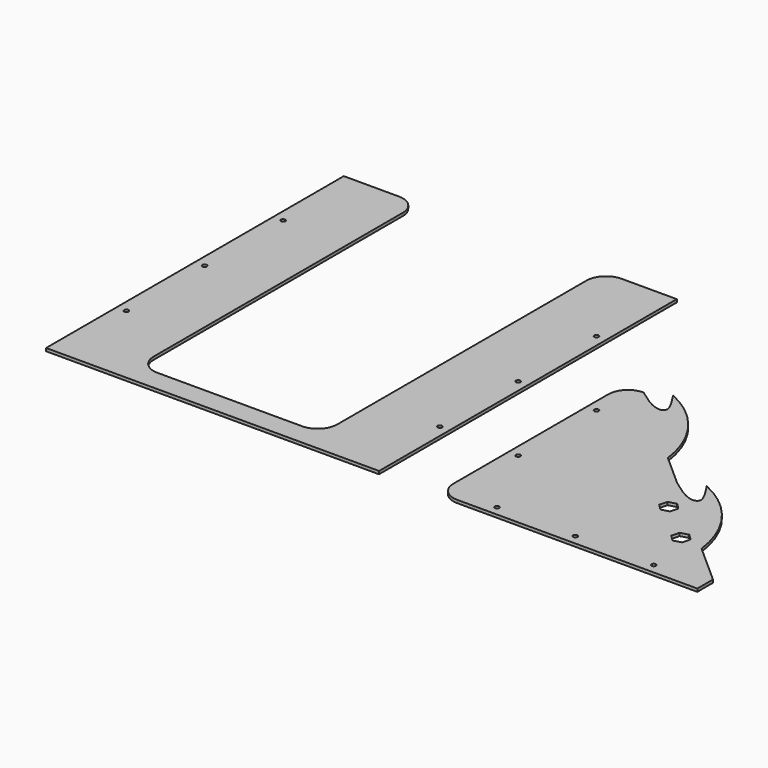
from build123d import *

# Parameters (mm, degrees)
F1_DEPTH   = 3
F2_D       = 4.5
F2_DEPTH   = 50
F2_TIP     = 1.3519363928
F2_2_D     = 4.5
F2_2_DEPTH = 50
F2_2_TIP   = 1.3519363928
F3_R       = 19.99999
F3_2_R     = 19.99999


# Not quite as in the source:
# - a fillet or chamfer is up to 0.001 mm smaller than in the source, because OpenCascade refuses the exact size


with BuildPart() as f1:
    # F0 (on Top) → F1 (new body)
    with BuildSketch(Plane.XY):
        Polygon((-40.9898807008, -128.9403379118), (-40.9898807008, 251.0596620882), (-117.2355602426, 251.0596620882), (-117.2355602426, -106.9403379118), (-304.744201159, -106.9403379118), (-304.744201159, 251.0596620882), (-380.9898807008, 251.0596620882), (-380.9898807008, -128.9403379118), align=None)
    extrude(amount=F1_DEPTH)

    # F2
    with Locations(Plane(origin=(0, 0, 0), x_dir=(1, 0, 0), z_dir=(0, 0, -1))):
        with Locations((29.0101192992, 38.9403379118), (71.5101192992, 118.9403379118), (29.0101192992, -61.0596620882), (29.0101192992, -161.0596620882), (71.5101192992, -241.0596620882), (151.5101192992, -241.0596620882), (231.5101192992, -241.0596620882), (151.5101192992, 118.9403379118), (231.5101192992, 118.9403379118), (-50.9898807008, -161.0596620882), (-50.9898807008, -61.0596620882), (-50.9898807008, 38.9403379118), (-370.9898807008, 38.9403379118), (-370.9898807008, -61.0596620882), (-370.9898807008, -161.0596620882)):
            Hole(F2_D / 2, depth=F2_DEPTH)
            with Locations((0, 0, -(F2_DEPTH + F2_TIP / 2))):  # 118° drill point
                Cone(0, F2_D / 2, F2_TIP, mode=Mode.SUBTRACT)

    # F3 (radius 20 in the source; OpenCascade refuses exactly that, so slightly less here)
    f3_edges = [f1.edges().sort_by_distance(p)[0] for p in [
        (-304.744201, -106.940338, 1.5),
        (-117.23556, -106.940338, 1.5),
        (-304.744201, 251.059662, 1.5),
        (-117.23556, 251.059662, 1.5),
    ]]
    fillet(f3_edges, radius=F3_R)


with BuildPart() as f1b:
    # F0 (on Top) → F1, piece 2 (new body)
    with BuildSketch(Plane.XY):
        with BuildLine():
            Line((39.0101192992, 108.6887940764), (19.0101192992, 108.6887940764))
            Line((19.0101192992, 108.6887940764), (19.0101192992, -128.9403379118))
            Line((19.0101192992, -128.9403379118), (284.0101192992, -128.9403379118))
            Line((284.0101192992, -128.9403379118), (284.0101192992, -108.9403379118))
            Line((284.0101192992, -108.9403379118), (243.4977915589, -72.953959459))
            ThreePointArc((243.4977915589, -72.953959459), (222.8255621797, -21.1730754944), (179.4192635913, 13.8196988242))
            add(Edge.make_bspline(
                [(157.8308492899, 3.1424580353), (178.8720103613, -13.0715758613), (192.9219916812, -13.2550713495), (191.4864058539, -4.0816277466), (179.4192635913, 13.8196988242)],
                knots=[0, 0, 0, 0, 0.5333043536, 1, 1, 1, 1], degree=3))
            Line((157.8308492899, 3.1424580353), (124.6770615683, 32.5923765821))
            ThreePointArc((124.6770615683, 32.5923765821), (104.0048321891, 84.3732605468), (60.5985336006, 119.3660348654))
            add(Edge.make_bspline(
                [(39.0101192992, 108.6887940764), (60.0512803706, 92.4747601798), (74.1012616905, 92.2912646916), (72.6656758632, 101.4647082946), (60.5985336006, 119.3660348654)],
                knots=[0, 0, 0, 0, 0.5333043536, 1, 1, 1, 1], degree=3))
        make_face()
        Polygon((183.7611458661, -38.6397473267), (175.7243851541, -40.7684827608), (169.8624658343, -34.872811537), (172.0373072265, -26.8484048792), (180.0740679385, -24.7196694452), (185.9359872583, -30.6153406689), align=None, mode=Mode.SUBTRACT)
        Polygon((212.7983209623, -62.6349506717), (220.8271718926, -60.3082533353), (226.856576358, -66.0980935359), (224.8571298931, -74.2146310729), (216.8282789629, -76.5413284094), (210.7988744974, -70.7514882088), align=None, mode=Mode.SUBTRACT)
    extrude(amount=F1_DEPTH)

    # F2#2
    with Locations(Plane(origin=(0, 0, 0), x_dir=(1, 0, 0), z_dir=(0, 0, -1))):
        with Locations((29.0101192992, 38.9403379118), (71.5101192992, 118.9403379118), (29.0101192992, -61.0596620882), (29.0101192992, -161.0596620882), (71.5101192992, -241.0596620882), (151.5101192992, -241.0596620882), (231.5101192992, -241.0596620882), (151.5101192992, 118.9403379118), (231.5101192992, 118.9403379118), (-50.9898807008, -161.0596620882), (-50.9898807008, -61.0596620882), (-50.9898807008, 38.9403379118), (-370.9898807008, 38.9403379118), (-370.9898807008, -61.0596620882), (-370.9898807008, -161.0596620882)):
            Hole(F2_2_D / 2, depth=F2_2_DEPTH)
            with Locations((0, 0, -(F2_2_DEPTH + F2_2_TIP / 2))):  # 118° drill point
                Cone(0, F2_2_D / 2, F2_2_TIP, mode=Mode.SUBTRACT)

    # F3#2 (radius 20 in the source; OpenCascade refuses exactly that, so slightly less here)
    f3_2_edges = [f1b.edges().sort_by_distance(p)[0] for p in [
        (19.010119, -128.940338, 1.5),
        (19.010119, 108.688794, 1.5),
    ]]
    fillet(f3_2_edges, radius=F3_2_R)


solid = Compound([f1.part, f1b.part])
